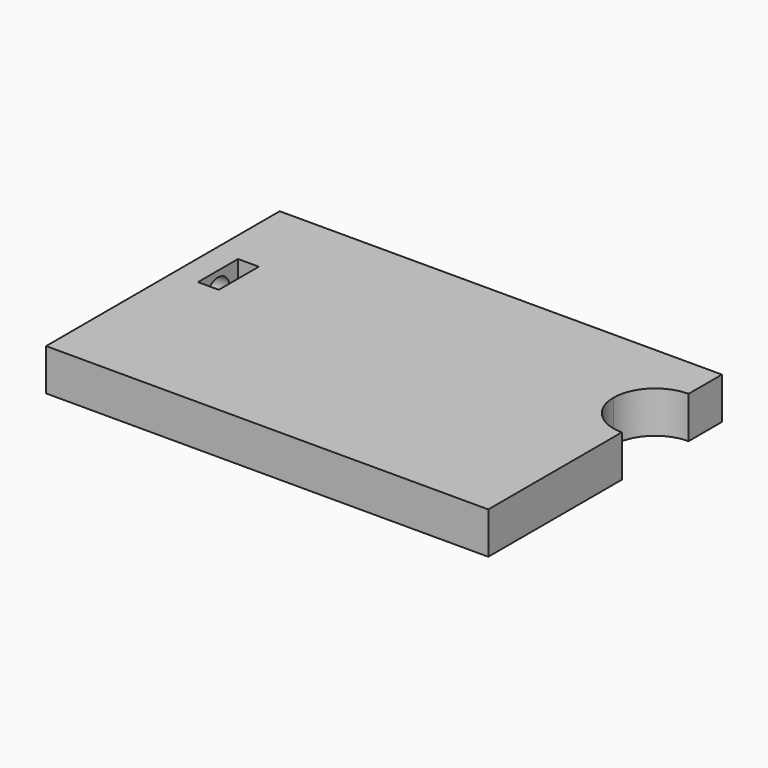
from build123d import *

# Parameters (mm, degrees)
F0_W     = 3
F0_H     = 10
F0_H_2   = 3
F1_DEPTH = 5
F2_R     = 1.75
F3_DEPTH = 20
F4_DEPTH = 20


# Not quite as in the source:
# - a feature names something its author has since deleted; it is built from what else it names


with BuildPart() as f1:
    # F0 (on Top) → F1 (new body)
    with BuildSketch(Plane.XY):
        with BuildLine():
            Line((-5, 25), (-47.5, 25))
            Line((-47.5, 25), (-47.5, 22))
            Line((-47.5, 22), (-47.5, 19))
            Line((-47.5, 19), (-50, 19))
            Line((-50, 19), (-50, 0))
            Line((-50, 0), (0, 0))
            Line((0, 0), (0, 20))
            ThreePointArc((0, 20), (-3.5355339059, 21.4644660941), (-5, 25))
        make_face()
        Polygon((-50, 22), (-53, 22), (-53, 0), (-50, 0), (-50, 19), align=None)
        with Locations((-51.5, 30)):
            Rectangle(F0_W, F0_H)
        with Locations((-51.5, 23.5)):
            Rectangle(F0_W, F0_H_2)
        with BuildLine():
            Line((0, 35), (-50, 35))
            Line((-50, 35), (-50, 25))
            Line((-50, 25), (-47.5, 25))
            Line((-47.5, 25), (-5, 25))
            ThreePointArc((-5, 25), (-3.5355339059, 28.5355339059), (0, 30))
            Line((0, 30), (0, 35))
        make_face()
    extrude(amount=F1_DEPTH)

    # F2 (on face) → F3 (cut)
    with BuildSketch(Plane(origin=(-53, 0, 0), x_dir=(0, -1, 0), z_dir=(-1, 0, 0))):
        with Locations((-22, 2.5274456161)):
            Circle(F2_R)
    extrude(amount=-F3_DEPTH, mode=Mode.SUBTRACT)

    # F2 (on face) → F4 (cut)
    with BuildSketch(Plane(origin=(-53, 0, 0), x_dir=(0, -1, 0), z_dir=(-1, 0, 0))):
        with BuildLine():
            ThreePointArc((22, 4.2774456161), (20.25, 2.5274456161), (22, 0.7774456161))
            Line((22, 0.7774456161), (22, 2.5274456161))
            Line((22, 2.5274456161), (22, 4.2774456161))
        make_face()
        with BuildLine():
            ThreePointArc((22, 0.7774456161), (23.2361299407, 1.2887032015), (23.7499961, 2.5237510221))
            Line((23.7499961, 2.5237510221), (22, 2.5274456161))
            Line((22, 2.5274456161), (22, 0.7774456161))
        make_face()
        with BuildLine():
            Line((22, 2.5274456161), (23.7499961, 2.5237510221))
            ThreePointArc((23.7499961, 2.5237510221), (23.749999025, 2.5255983181), (23.75, 2.5274456161))
            ThreePointArc((23.75, 2.5274456161), (23.2374368671, 3.7648824831), (22, 4.2774456161))
            Line((22, 4.2774456161), (22, 2.5274456161))
        make_face()
    extrude(amount=-F4_DEPTH, mode=Mode.SUBTRACT)


solid = f1.part
